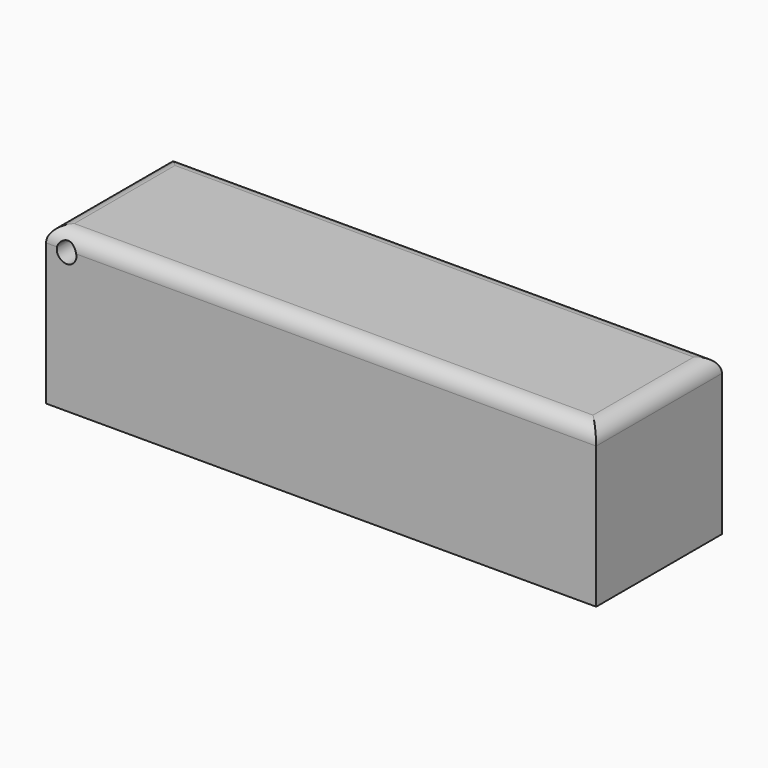
from build123d import *

# Parameters (mm, degrees)
F0_W        = 50.8
F0_H        = 50.8
F1_DEPTH    = 50.8
F2_DEPTH    = 127
F4_D        = 6.35
F5_T1_DEPTH = 76.2
F5_T3_DEPTH = 203.2


# Not quite as in the source:
# - a fillet or chamfer that OpenCascade refuses, or shapes differently, is made with other operations: its cross-section is extruded or revolved along the edge and cut away or added


with BuildPart() as f1:
    # F0 (on Front) → F1 (new body)
    with BuildSketch(Plane.XZ):
        Rectangle(F0_W, F0_H)
    extrude(amount=F1_DEPTH)

    # F2 (add): a face of the model
    f2_faces = [f1.faces().sort_by_distance(p)[0] for p in [
        (25.4, -25.4, 0),
    ]]
    extrude(f2_faces, amount=F2_DEPTH)

    # F4 (through all)
    with Locations(Plane.XZ.offset(50.8)):
        with Locations((-18.774760887, 19.6526572108)):
            Hole(F4_D / 2)

    # F5: fillet of radius 5.08 on 4 edges, made by hand

    # F5_s2 → F5_t1 (cut)
    with BuildSketch(Plane.XZ.offset(-12.7)):
        with BuildLine():
            ThreePointArc((-25.4, 20.32), (-23.9121024484, 23.9121024484), (-20.32, 25.4))
            Line((-20.32, 25.4), (-25.4, 25.4))
            Line((-25.4, 25.4), (-25.4, 20.32))
        make_face()
        with BuildLine():
            ThreePointArc((152.4, 20.32), (150.9121024484, 23.9121024484), (147.32, 25.4))
            Line((147.32, 25.4), (152.4, 25.4))
            Line((152.4, 25.4), (152.4, 20.32))
        make_face()
    extrude(amount=F5_T1_DEPTH, mode=Mode.SUBTRACT)

    # F5_s4 → F5_t3 (cut)
    with BuildSketch(Plane.YZ.offset(-38.1)):
        with BuildLine():
            ThreePointArc((0, 20.32), (-1.4878975516, 23.9121024484), (-5.08, 25.4))
            Line((-5.08, 25.4), (0, 25.4))
            Line((0, 25.4), (0, 20.32))
        make_face()
        with BuildLine():
            ThreePointArc((-50.8, 20.32), (-49.3121024484, 23.9121024484), (-45.72, 25.4))
            Line((-45.72, 25.4), (-50.8, 25.4))
            Line((-50.8, 25.4), (-50.8, 20.32))
        make_face()
    extrude(amount=F5_T3_DEPTH, mode=Mode.SUBTRACT)


solid = f1.part
